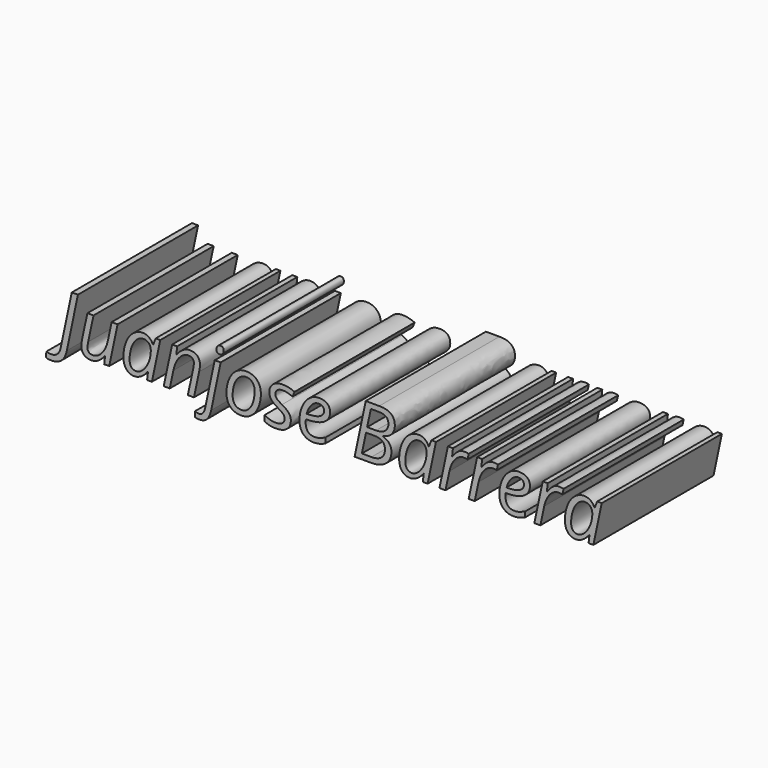
from build123d import *

# Parameters (mm, degrees)
F0_TEXT_SIZE = 12.4797289674
F1_DEPTH     = 25.4


# Not quite as in the source:
# - Text() gives the source's letters only with a copy of the font that has no kerning and outlines rounded to 1/6400 em; it was checked with that copy


with BuildPart() as f1:
    # F0 (on Front) → F1 (new body)
    with BuildSketch(Plane.XZ):
        with Locations((-47.6671282619, 0)):
            Text('Juanjose Barrera', F0_TEXT_SIZE, font='Open Sans', font_style=FontStyle.ITALIC, text_align=(TextAlign.LEFT, TextAlign.BOTTOM))
    extrude(amount=F1_DEPTH)


solid = f1.part
